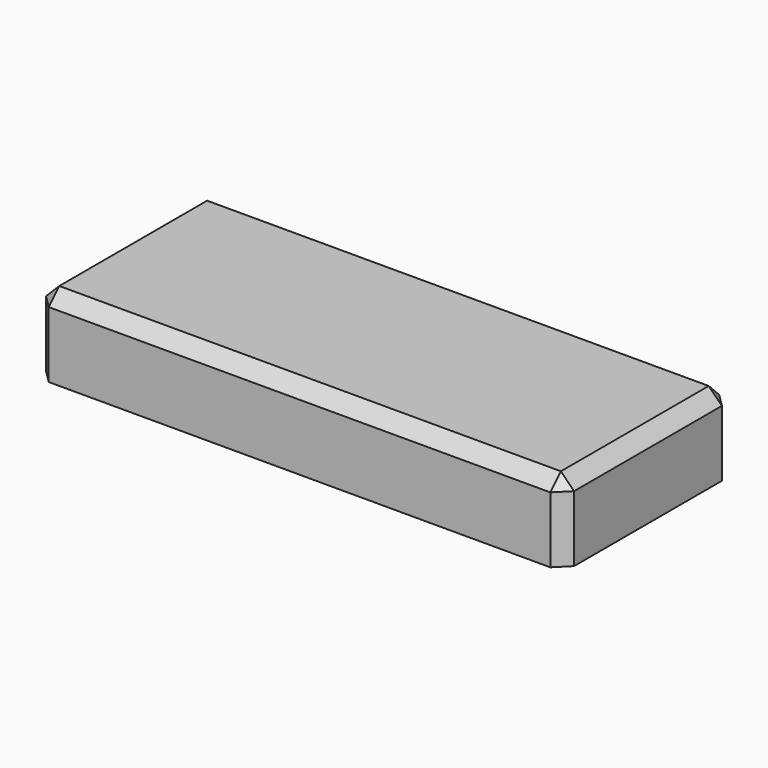
from build123d import *

# Parameters (mm, degrees)
F0_W     = 200
F0_H     = 30
F1_DEPTH = 80
F2_T     = -10
F3_R     = 10
F4_SIZE  = 5


with BuildPart() as f1:
    # F0 (on Front) → F1 (new body)
    with BuildSketch(Plane.XZ):
        Rectangle(F0_W, F0_H)
    extrude(amount=-F1_DEPTH)

    # F2
    f2_openings = [f1.faces().sort_by_distance(p)[0] for p in [
        (0, 40, -15),
    ]]
    offset(amount=F2_T, openings=f2_openings)

    # F3
    f3_edges = [f1.edges().sort_by_distance(p)[0] for p in [
        (-90, 10, -5),
        (0, 10, 5),
        (-90, 40, 5),
        (90, 10, -5),
        (90, 40, 5),
        (90, 70, -5),
        (0, 70, 5),
        (-90, 70, -5),
    ]]
    fillet(f3_edges, radius=F3_R)

    # F4
    f4_edges = [f1.edges().sort_by_distance(p)[0] for p in [
        (-100, 0, 0),
        (0, 0, 15),
        (-100, 40, 15),
        (-100, 80, 0),
        (0, 80, 15),
        (100, 80, 0),
        (100, 40, 15),
        (100, 0, 0),
    ]]
    chamfer(f4_edges, length=F4_SIZE)


solid = f1.part
